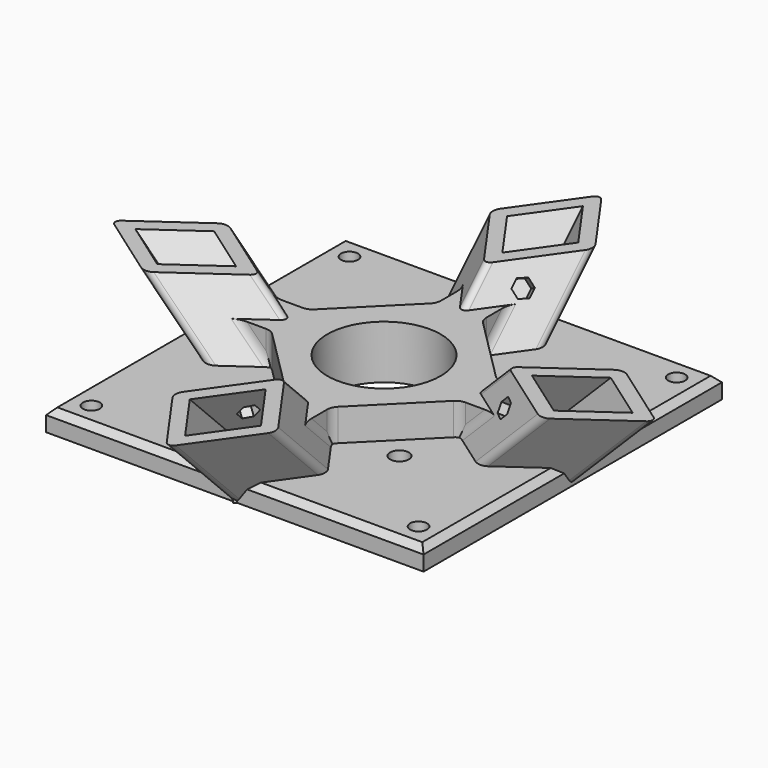
from build123d import *

# Parameters (mm, degrees)
F1_DEPTH      = 4.318
F9_DEPTH      = 2.54
F10_COUNT     = 4
F10_ANGLE     = 270
F14_DEPTH     = 10.795
F23_W         = 111.76
F23_H         = 15.24
F24_DEPTH     = 152.4
F25_T4_DEPTH  = 14.9351248517
F25_T9_DEPTH  = 24.0949860952
F25_T14_DEPTH = 30.2015602576
F25_T19_DEPTH = 30.2015602576
F25_T24_DEPTH = 24.0949860952
F25_T29_DEPTH = 24.0949860952
F25_T34_DEPTH = 30.2015602576
F25_T39_DEPTH = 30.2015602576
F25_T44_DEPTH = 24.0949860952
F25_T49_DEPTH = 14.9351248517
F26_T4_DEPTH  = 24.0949860952
F26_T9_DEPTH  = 30.2015602576
F26_T14_DEPTH = 30.2015602576
F26_T19_DEPTH = 24.0949860952
F26_T24_DEPTH = 14.9351248517
F26_T29_DEPTH = 14.9351248517
F26_T34_DEPTH = 24.0949860952
F26_T39_DEPTH = 24.0949860952
F26_T44_DEPTH = 30.2015602576
F26_T49_DEPTH = 30.2015602576
F27_T1_DEPTH  = 9.1072561211
F27_T6_DEPTH  = 14.4203734854
F27_T11_DEPTH = 14.4203734856
F27_T16_DEPTH = 14.4203734854
F27_T21_DEPTH = 14.4203734856
F27_T26_DEPTH = 14.4203734854
F27_T31_DEPTH = 14.4203734856
F27_T36_DEPTH = 14.4203734856
F27_T41_DEPTH = 14.4203734854
F28_W         = 76.2
F28_H         = 75.2855999997
F29_DEPTH     = 4.318
F15_R         = 1.905
F30_DEPTH     = 25.4
F12_R         = 11.43
F31_DEPTH     = 25.4
F32_R         = 1.7145
F33_DEPTH     = 4.318
F34_SIZE      = 1.27


# Not quite as in the source:
# - a fillet or chamfer that OpenCascade refuses, or shapes differently, is made with other operations: its cross-section is extruded or revolved along the edge and cut away or added


with BuildPart() as f1:
    # F0 (on Top) → F1 (new body)
    with BuildSketch(Plane.XY):
        Polygon((38.1, 0), (0, 38.1), (-38.1, 0), (0, -38.1), align=None)
    extrude(amount=F1_DEPTH)

    # F5 (on offset) → F6 (join, up to the next surface of F1)
    with BuildSketch(Plane(origin=(0, -35.9210244843, 35.9210244843), x_dir=(1, 0, 0), z_dir=(0, 0.7071067812, -0.7071067812))):
        Polygon((10.5607811984, 16.3799871648), (0, 26.9407683632), (-10.5607811984, 16.3799871648), (0, 5.8192059665), align=None)
        Polygon((-7.1842048969, 16.3799871648), (0, 23.5641920617), (7.1842048969, 16.3799871648), (0, 9.195782268), align=None, mode=Mode.SUBTRACT)
    extrude(until=Until.NEXT)

    # F8 (on offset) → F9 (cut)
    with BuildSketch(Plane(origin=(2.9096029833, -2.0574, -2.0574), x_dir=(-0.4082482905, -0.8660254038, 0.2886751346), z_dir=(-0.7071067812, 0.5, 0.5))):
        Polygon((30.7118833173, 5.5090421757), (32.268461045, 6.6097088424), (32.0935446144, 8.5080780308), (30.3620504561, 9.3057805526), (28.8054727285, 8.2051138859), (28.9803891591, 6.3067446975), align=None)
    extrude(amount=-F9_DEPTH, mode=Mode.SUBTRACT)


with BuildPart() as f10_1:
    # F10: instance of F1
    add(f1.part.rotate(Axis((0, 0, 13.9133725866), (0, 0, 1)), 1 * F10_ANGLE / (F10_COUNT - 1)))


with BuildPart() as f10_2:
    # F10: instance of F1
    add(f1.part.rotate(Axis((0, 0, 13.9133725866), (0, 0, 1)), 2 * F10_ANGLE / (F10_COUNT - 1)))


with BuildPart() as f10_3:
    # F10: instance of F1
    add(f1.part.rotate(Axis((0, 0, 13.9133725866), (0, 0, 1)), 3 * F10_ANGLE / (F10_COUNT - 1)))


with BuildPart() as f14:
    # F13 (on Top) → F14 (new body)
    with BuildSketch(Plane.XY):
        Polygon((19.05, 4.597891134), (4.5978911339, 19.05), (-4.5978911339, 19.05), (-19.05, 4.5978911339), (-19.05, -4.597891134), (-4.5978911339, -19.05), (4.597891134, -19.05), (19.05, -4.5978911339), align=None)
    extrude(amount=F14_DEPTH)


with BuildPart() as f10_2_1:
    add(f10_2.part)

    # F16: union F14
    add(f14.part)

    # F17: union F10_3, F1, F10_1
    add(f10_3.part)
    add(f1.part)
    add(f10_1.part)

    # F17_face (on face) → F18 (join, up to the next surface of F10_2)
    with BuildSketch(Plane(origin=(-19.05, 3.0712475933, 8.6360000001), x_dir=(0, -1, 0), z_dir=(-1, 0, 0))):
        Polygon((3.0532870811, 2.1589999999), (-1.5266435405, 2.1589999999), (-1.5266435405, -4.3180000001), align=None)
        Polygon((7.6691387273, -4.3180000001), (7.6691387273, 2.1589999999), (3.0892081056, 2.1589999999), align=None)
    extrude(until=Until.NEXT)

    # F16_face (on face) → F19 (join, up to the next surface of F10_2)
    with BuildSketch(Plane(origin=(-3.0712475933, 19.05, 8.6359999999), x_dir=(-1, 0, 0), z_dir=(0, 1, 0))):
        Polygon((1.5266435406, -4.3179999999), (1.5266435406, 2.1590000001), (-3.0532870811, 2.1590000001), align=None)
        Polygon((-7.6691387272, -4.3179999998), (-3.0892081056, 2.1590000001), (-7.6691387272, 2.1590000001), align=None)
    extrude(until=Until.NEXT)

    # F17_face1 (on face) → F20 (join, up to the next surface of F10_2)
    with BuildSketch(Plane(origin=(19.05, -3.0712475933, 8.6360000001), x_dir=(0, 1, 0), z_dir=(1, 0, 0))):
        Polygon((3.0532870811, 2.1589999999), (-1.5266435405, 2.1589999999), (-1.5266435405, -4.3180000001), align=None)
        Polygon((7.6691387273, -4.3180000001), (7.6691387273, 2.1589999999), (3.0892081056, 2.1589999999), align=None)
    extrude(until=Until.NEXT)

    # F17_face2 (on face) → F21 (join, up to the next surface of F10_2)
    with BuildSketch(Plane(origin=(3.0712475934, -19.05, 8.636), x_dir=(1, 0, 0), z_dir=(0, -1, 0))):
        Polygon((1.5266435406, -4.318), (1.5266435406, 2.159), (-3.0532870811, 2.159), align=None)
        Polygon((-3.0892081056, 2.159), (-7.6691387273, 2.159), (-7.6691387273, -4.318), align=None)
    extrude(until=Until.NEXT)

    # F23 (on offset) → F24 (cut)
    with BuildSketch(Plane.YZ.offset(63.5)):
        with Locations((0, 24.4856)):
            Rectangle(F23_W, F23_H)
    extrude(amount=-F24_DEPTH, mode=Mode.SUBTRACT)

    # F25: fillet of radius 1.27 on 8 edges, made by hand


with BuildPart() as f25_tool2:
    # F25_s3 → F25_t4 (new body)
    with BuildSketch(Plane(origin=(0, 23.2254640303, 23.2254640303), x_dir=(1, 0, 0), z_dir=(0, -0.7071067812, -0.7071067812))):
        with BuildLine():
            ThreePointArc((0.8980256121, -6.7172315786), (0, -6.3452571907), (-0.8980256121, -6.7172315786))
            Line((-0.8980256121, -6.7172315786), (0, -5.8192059665))
            Line((0, -5.8192059665), (0.8980256121, -6.7172315786))
        make_face()
    extrude(amount=F25_T4_DEPTH)

    split(bisect_by=Plane.XY.offset(10.795), keep=Keep.TOP)


with BuildPart() as f10_2_2:
    add(f10_2_1.part)

    # F25_t1: cut F25_tool2
    add(f25_tool2.part, mode=Mode.SUBTRACT)


with BuildPart() as f25_tool7:
    # F25_s8 → F25_t9 (new body)
    with BuildSketch(Plane(origin=(0, 30.6930640303, 30.6930640303), x_dir=(1, 0, 0), z_dir=(0, -0.7071067812, -0.7071067812))):
        with BuildLine():
            ThreePointArc((9.6627555863, -17.2780127769), (10.0347299742, -16.3799871648), (9.6627555863, -15.4819615527))
            Line((9.6627555863, -15.4819615527), (10.5607811984, -16.3799871648))
            Line((10.5607811984, -16.3799871648), (9.6627555863, -17.2780127769))
        make_face()
    extrude(amount=F25_T9_DEPTH)

    split(bisect_by=Plane.XY.offset(4.318), keep=Keep.TOP)


with BuildPart() as f10_2_3:
    add(f10_2_2.part)

    # F25_t6: cut F25_tool7
    add(f25_tool7.part, mode=Mode.SUBTRACT)


with BuildPart() as f25_tool12:
    # F25_s13 → F25_t14 (new body)
    with BuildSketch(Plane(origin=(0, 38.1606640303, 38.1606640303), x_dir=(1, 0, 0), z_dir=(0, -0.7071067812, -0.7071067812))):
        with BuildLine():
            ThreePointArc((0.8980256121, -26.0427427511), (0, -26.414717139), (-0.8980256121, -26.0427427511))
            Line((-0.8980256121, -26.0427427511), (0, -26.9407683632))
            Line((0, -26.9407683632), (0.8980256121, -26.0427427511))
        make_face()
    extrude(amount=F25_T14_DEPTH)

    split(bisect_by=Plane(origin=(-19.05, 19.05, 0), x_dir=(0, 0, 1), z_dir=(-0.7071067812, 0.7071067812, 0)), keep=Keep.TOP)


with BuildPart() as f10_2_4:
    add(f10_2_3.part)

    # F25_t11: cut F25_tool12
    add(f25_tool12.part, mode=Mode.SUBTRACT)


with BuildPart() as f25_tool17:
    # F25_s18 → F25_t19 (new body)
    with BuildSketch(Plane(origin=(0, 38.1606640303, 38.1606640303), x_dir=(1, 0, 0), z_dir=(0, -0.7071067812, -0.7071067812))):
        with BuildLine():
            ThreePointArc((0.8980256121, -26.0427427511), (0, -26.414717139), (-0.8980256121, -26.0427427511))
            Line((-0.8980256121, -26.0427427511), (0, -26.9407683632))
            Line((0, -26.9407683632), (0.8980256121, -26.0427427511))
        make_face()
    extrude(amount=F25_T19_DEPTH)

    split(bisect_by=Plane(origin=(19.05, 19.05, 0), x_dir=(0, 0, 1), z_dir=(0.7071067812, 0.7071067812, 0)), keep=Keep.TOP)


with BuildPart() as f10_2_5:
    add(f10_2_4.part)

    # F25_t16: cut F25_tool17
    add(f25_tool17.part, mode=Mode.SUBTRACT)


with BuildPart() as f25_tool22:
    # F25_s23 → F25_t24 (new body)
    with BuildSketch(Plane(origin=(0, 30.6930640303, 30.6930640303), x_dir=(1, 0, 0), z_dir=(0, -0.7071067812, -0.7071067812))):
        with BuildLine():
            ThreePointArc((-9.6627555863, -17.2780127769), (-10.0347299742, -16.3799871648), (-9.6627555863, -15.4819615527))
            Line((-9.6627555863, -15.4819615527), (-10.5607811984, -16.3799871648))
            Line((-10.5607811984, -16.3799871648), (-9.6627555863, -17.2780127769))
        make_face()
    extrude(amount=F25_T24_DEPTH)

    split(bisect_by=Plane.XY.offset(4.318), keep=Keep.TOP)


with BuildPart() as f10_2_6:
    add(f10_2_5.part)

    # F25_t21: cut F25_tool22
    add(f25_tool22.part, mode=Mode.SUBTRACT)


with BuildPart() as f25_tool27:
    # F25_s28 → F25_t29 (new body)
    with BuildSketch(Plane(origin=(30.6930640303, 0, 30.6930640303), x_dir=(0, 1, 0), z_dir=(-0.7071067812, 0, -0.7071067812))):
        with BuildLine():
            ThreePointArc((9.6627555863, 17.2780127769), (10.0347299742, 16.3799871648), (9.6627555863, 15.4819615527))
            Line((9.6627555863, 15.4819615527), (10.5607811984, 16.3799871648))
            Line((10.5607811984, 16.3799871648), (9.6627555863, 17.2780127769))
        make_face()
    extrude(amount=F25_T29_DEPTH)

    split(bisect_by=Plane.XY.offset(4.318), keep=Keep.TOP)


with BuildPart() as f10_2_7:
    add(f10_2_6.part)

    # F25_t26: cut F25_tool27
    add(f25_tool27.part, mode=Mode.SUBTRACT)


with BuildPart() as f25_tool32:
    # F25_s33 → F25_t34 (new body)
    with BuildSketch(Plane(origin=(38.1606640303, 0, 38.1606640303), x_dir=(0, 1, 0), z_dir=(-0.7071067812, 0, -0.7071067812))):
        with BuildLine():
            ThreePointArc((-0.8980256121, 26.0427427511), (0, 26.414717139), (0.8980256121, 26.0427427511))
            Line((0.8980256121, 26.0427427511), (0, 26.9407683632))
            Line((0, 26.9407683632), (-0.8980256121, 26.0427427511))
        make_face()
    extrude(amount=F25_T34_DEPTH)

    split(bisect_by=Plane(origin=(19.05, 19.05, 0), x_dir=(0, 0, 1), z_dir=(0.7071067812, 0.7071067812, 0)), keep=Keep.TOP)


with BuildPart() as f10_2_8:
    add(f10_2_7.part)

    # F25_t31: cut F25_tool32
    add(f25_tool32.part, mode=Mode.SUBTRACT)


with BuildPart() as f25_tool37:
    # F25_s38 → F25_t39 (new body)
    with BuildSketch(Plane(origin=(38.1606640303, 0, 38.1606640303), x_dir=(0, 1, 0), z_dir=(-0.7071067812, 0, -0.7071067812))):
        with BuildLine():
            ThreePointArc((-0.8980256121, 26.0427427511), (0, 26.414717139), (0.8980256121, 26.0427427511))
            Line((0.8980256121, 26.0427427511), (0, 26.9407683632))
            Line((0, 26.9407683632), (-0.8980256121, 26.0427427511))
        make_face()
    extrude(amount=F25_T39_DEPTH)

    split(bisect_by=Plane(origin=(19.05, -19.05, 0), x_dir=(0, 0, 1), z_dir=(0.7071067812, -0.7071067812, 0)), keep=Keep.TOP)


with BuildPart() as f10_2_9:
    add(f10_2_8.part)

    # F25_t36: cut F25_tool37
    add(f25_tool37.part, mode=Mode.SUBTRACT)


with BuildPart() as f25_tool42:
    # F25_s43 → F25_t44 (new body)
    with BuildSketch(Plane(origin=(30.6930640303, 0, 30.6930640303), x_dir=(0, 1, 0), z_dir=(-0.7071067812, 0, -0.7071067812))):
        with BuildLine():
            ThreePointArc((-9.6627555863, 17.2780127769), (-10.0347299742, 16.3799871648), (-9.6627555863, 15.4819615527))
            Line((-9.6627555863, 15.4819615527), (-10.5607811984, 16.3799871648))
            Line((-10.5607811984, 16.3799871648), (-9.6627555863, 17.2780127769))
        make_face()
    extrude(amount=F25_T44_DEPTH)

    split(bisect_by=Plane.XY.offset(4.318), keep=Keep.TOP)


with BuildPart() as f10_2_10:
    add(f10_2_9.part)

    # F25_t41: cut F25_tool42
    add(f25_tool42.part, mode=Mode.SUBTRACT)


with BuildPart() as f25_tool47:
    # F25_s48 → F25_t49 (new body)
    with BuildSketch(Plane(origin=(23.2254640303, 0, 23.2254640303), x_dir=(0, 1, 0), z_dir=(-0.7071067812, 0, -0.7071067812))):
        with BuildLine():
            ThreePointArc((-0.8980256121, 6.7172315786), (0, 6.3452571907), (0.8980256121, 6.7172315786))
            Line((0.8980256121, 6.7172315786), (0, 5.8192059665))
            Line((0, 5.8192059665), (-0.8980256121, 6.7172315786))
        make_face()
    extrude(amount=F25_T49_DEPTH)

    split(bisect_by=Plane.XY.offset(10.795), keep=Keep.TOP)


with BuildPart() as f10_2_11:
    add(f10_2_10.part)

    # F25_t46: cut F25_tool47
    add(f25_tool47.part, mode=Mode.SUBTRACT)

    # F26: fillet of radius 1.27 on 8 edges, made by hand


with BuildPart() as f26_tool2:
    # F26_s3 → F26_t4 (new body)
    with BuildSketch(Plane(origin=(0, -30.6930640303, 30.6930640303), x_dir=(1, 0, 0), z_dir=(0, 0.7071067812, -0.7071067812))):
        with BuildLine():
            ThreePointArc((-9.6627555863, 17.2780127769), (-10.0347299742, 16.3799871648), (-9.6627555863, 15.4819615527))
            Line((-9.6627555863, 15.4819615527), (-10.5607811984, 16.3799871648))
            Line((-10.5607811984, 16.3799871648), (-9.6627555863, 17.2780127769))
        make_face()
    extrude(amount=F26_T4_DEPTH)

    split(bisect_by=Plane.XY.offset(4.318), keep=Keep.TOP)


with BuildPart() as f10_2_12:
    add(f10_2_11.part)

    # F26_t1: cut F26_tool2
    add(f26_tool2.part, mode=Mode.SUBTRACT)


with BuildPart() as f26_tool7:
    # F26_s8 → F26_t9 (new body)
    with BuildSketch(Plane(origin=(0, -38.1606640303, 38.1606640303), x_dir=(1, 0, 0), z_dir=(0, 0.7071067812, -0.7071067812))):
        with BuildLine():
            ThreePointArc((0.8980256121, 26.0427427511), (0, 26.414717139), (-0.8980256121, 26.0427427511))
            Line((-0.8980256121, 26.0427427511), (0, 26.9407683632))
            Line((0, 26.9407683632), (0.8980256121, 26.0427427511))
        make_face()
    extrude(amount=F26_T9_DEPTH)

    split(bisect_by=Plane(origin=(-19.05, -19.05, 0), x_dir=(0, 0, 1), z_dir=(-0.7071067812, -0.7071067812, 0)), keep=Keep.TOP)


with BuildPart() as f10_2_13:
    add(f10_2_12.part)

    # F26_t6: cut F26_tool7
    add(f26_tool7.part, mode=Mode.SUBTRACT)


with BuildPart() as f26_tool12:
    # F26_s13 → F26_t14 (new body)
    with BuildSketch(Plane(origin=(0, -38.1606640303, 38.1606640303), x_dir=(1, 0, 0), z_dir=(0, 0.7071067812, -0.7071067812))):
        with BuildLine():
            ThreePointArc((0.8980256121, 26.0427427511), (0, 26.414717139), (-0.8980256121, 26.0427427511))
            Line((-0.8980256121, 26.0427427511), (0, 26.9407683632))
            Line((0, 26.9407683632), (0.8980256121, 26.0427427511))
        make_face()
    extrude(amount=F26_T14_DEPTH)

    split(bisect_by=Plane(origin=(19.05, -19.05, 0), x_dir=(0, 0, 1), z_dir=(0.7071067812, -0.7071067812, 0)), keep=Keep.TOP)


with BuildPart() as f10_2_14:
    add(f10_2_13.part)

    # F26_t11: cut F26_tool12
    add(f26_tool12.part, mode=Mode.SUBTRACT)


with BuildPart() as f26_tool17:
    # F26_s18 → F26_t19 (new body)
    with BuildSketch(Plane(origin=(0, -30.6930640303, 30.6930640303), x_dir=(1, 0, 0), z_dir=(0, 0.7071067812, -0.7071067812))):
        with BuildLine():
            ThreePointArc((9.6627555863, 17.2780127769), (10.0347299742, 16.3799871648), (9.6627555863, 15.4819615527))
            Line((9.6627555863, 15.4819615527), (10.5607811984, 16.3799871648))
            Line((10.5607811984, 16.3799871648), (9.6627555863, 17.2780127769))
        make_face()
    extrude(amount=F26_T19_DEPTH)

    split(bisect_by=Plane.XY.offset(4.318), keep=Keep.TOP)


with BuildPart() as f10_2_15:
    add(f10_2_14.part)

    # F26_t16: cut F26_tool17
    add(f26_tool17.part, mode=Mode.SUBTRACT)


with BuildPart() as f26_tool22:
    # F26_s23 → F26_t24 (new body)
    with BuildSketch(Plane(origin=(0, -23.2254640303, 23.2254640303), x_dir=(1, 0, 0), z_dir=(0, 0.7071067812, -0.7071067812))):
        with BuildLine():
            ThreePointArc((0.8980256121, 6.7172315786), (0, 6.3452571907), (-0.8980256121, 6.7172315786))
            Line((-0.8980256121, 6.7172315786), (0, 5.8192059665))
            Line((0, 5.8192059665), (0.8980256121, 6.7172315786))
        make_face()
    extrude(amount=F26_T24_DEPTH)

    split(bisect_by=Plane.XY.offset(10.795), keep=Keep.TOP)


with BuildPart() as f10_2_16:
    add(f10_2_15.part)

    # F26_t21: cut F26_tool22
    add(f26_tool22.part, mode=Mode.SUBTRACT)


with BuildPart() as f26_tool27:
    # F26_s28 → F26_t29 (new body)
    with BuildSketch(Plane(origin=(-23.2254640303, 0, 23.2254640303), x_dir=(0, 1, 0), z_dir=(0.7071067812, 0, -0.7071067812))):
        with BuildLine():
            ThreePointArc((0.8980256121, -6.7172315786), (0, -6.3452571907), (-0.8980256121, -6.7172315786))
            Line((-0.8980256121, -6.7172315786), (0, -5.8192059665))
            Line((0, -5.8192059665), (0.8980256121, -6.7172315786))
        make_face()
    extrude(amount=F26_T29_DEPTH)

    split(bisect_by=Plane.XY.offset(10.795), keep=Keep.TOP)


with BuildPart() as f10_2_17:
    add(f10_2_16.part)

    # F26_t26: cut F26_tool27
    add(f26_tool27.part, mode=Mode.SUBTRACT)


with BuildPart() as f26_tool32:
    # F26_s33 → F26_t34 (new body)
    with BuildSketch(Plane(origin=(-30.6930640303, 0, 30.6930640303), x_dir=(0, 1, 0), z_dir=(0.7071067812, 0, -0.7071067812))):
        with BuildLine():
            ThreePointArc((-9.6627555863, -17.2780127769), (-10.0347299742, -16.3799871648), (-9.6627555863, -15.4819615527))
            Line((-9.6627555863, -15.4819615527), (-10.5607811984, -16.3799871648))
            Line((-10.5607811984, -16.3799871648), (-9.6627555863, -17.2780127769))
        make_face()
    extrude(amount=F26_T34_DEPTH)

    split(bisect_by=Plane.XY.offset(4.318), keep=Keep.TOP)


with BuildPart() as f10_2_18:
    add(f10_2_17.part)

    # F26_t31: cut F26_tool32
    add(f26_tool32.part, mode=Mode.SUBTRACT)


with BuildPart() as f26_tool37:
    # F26_s38 → F26_t39 (new body)
    with BuildSketch(Plane(origin=(-30.6930640303, 0, 30.6930640303), x_dir=(0, 1, 0), z_dir=(0.7071067812, 0, -0.7071067812))):
        with BuildLine():
            ThreePointArc((9.6627555863, -17.2780127769), (10.0347299742, -16.3799871648), (9.6627555863, -15.4819615527))
            Line((9.6627555863, -15.4819615527), (10.5607811984, -16.3799871648))
            Line((10.5607811984, -16.3799871648), (9.6627555863, -17.2780127769))
        make_face()
    extrude(amount=F26_T39_DEPTH)

    split(bisect_by=Plane.XY.offset(4.318), keep=Keep.TOP)


with BuildPart() as f10_2_19:
    add(f10_2_18.part)

    # F26_t36: cut F26_tool37
    add(f26_tool37.part, mode=Mode.SUBTRACT)


with BuildPart() as f26_tool42:
    # F26_s43 → F26_t44 (new body)
    with BuildSketch(Plane(origin=(-38.1606640303, 0, 38.1606640303), x_dir=(0, 1, 0), z_dir=(0.7071067812, 0, -0.7071067812))):
        with BuildLine():
            ThreePointArc((0.8980256121, -26.0427427511), (0, -26.414717139), (-0.8980256121, -26.0427427511))
            Line((-0.8980256121, -26.0427427511), (0, -26.9407683632))
            Line((0, -26.9407683632), (0.8980256121, -26.0427427511))
        make_face()
    extrude(amount=F26_T44_DEPTH)

    split(bisect_by=Plane(origin=(-19.05, -19.05, 0), x_dir=(0, 0, 1), z_dir=(-0.7071067812, -0.7071067812, 0)), keep=Keep.TOP)


with BuildPart() as f10_2_20:
    add(f10_2_19.part)

    # F26_t41: cut F26_tool42
    add(f26_tool42.part, mode=Mode.SUBTRACT)


with BuildPart() as f26_tool47:
    # F26_s48 → F26_t49 (new body)
    with BuildSketch(Plane(origin=(-38.1606640303, 0, 38.1606640303), x_dir=(0, 1, 0), z_dir=(0.7071067812, 0, -0.7071067812))):
        with BuildLine():
            ThreePointArc((0.8980256121, -26.0427427511), (0, -26.414717139), (-0.8980256121, -26.0427427511))
            Line((-0.8980256121, -26.0427427511), (0, -26.9407683632))
            Line((0, -26.9407683632), (0.8980256121, -26.0427427511))
        make_face()
    extrude(amount=F26_T49_DEPTH)

    split(bisect_by=Plane(origin=(-19.05, 19.05, 0), x_dir=(0, 0, 1), z_dir=(-0.7071067812, 0.7071067812, 0)), keep=Keep.TOP)


with BuildPart() as f10_2_21:
    add(f10_2_20.part)

    # F26_t46: cut F26_tool47
    add(f26_tool47.part, mode=Mode.SUBTRACT)

    # F27: fillet of radius 2.54 on 16 edges, made by hand

    # F27_s2 → F27_t1 (join)
    with BuildSketch(Plane.XY.offset(1.6877438789)):
        with BuildLine():
            ThreePointArc((18.3060512242, 5.3418399098), (19.1300865302, 4.7912371214), (20.1021024484, 4.597891134))
            Line((20.1021024484, 4.597891134), (19.05, 4.597891134))
            Line((19.05, 4.597891134), (18.3060512242, 5.3418399098))
        make_face()
        with BuildLine():
            ThreePointArc((4.5978911339, 20.1021024484), (4.7912371213, 19.1300865302), (5.3418399097, 18.3060512242))
            Line((5.3418399097, 18.3060512242), (4.5978911339, 19.05))
            Line((4.5978911339, 19.05), (4.5978911339, 20.1021024484))
        make_face()
        with BuildLine():
            ThreePointArc((-5.3418399097, 18.3060512242), (-4.7912371213, 19.1300865302), (-4.5978911339, 20.1021024484))
            Line((-4.5978911339, 20.1021024484), (-4.5978911339, 19.05))
            Line((-4.5978911339, 19.05), (-5.3418399097, 18.3060512242))
        make_face()
        with BuildLine():
            ThreePointArc((-20.1021024484, 4.5978911339), (-19.1300865302, 4.7912371213), (-18.3060512242, 5.3418399097))
            Line((-18.3060512242, 5.3418399097), (-19.05, 4.5978911339))
            Line((-19.05, 4.5978911339), (-20.1021024484, 4.5978911339))
        make_face()
        with BuildLine():
            ThreePointArc((-18.3060512242, -5.3418399097), (-19.1300865302, -4.7912371214), (-20.1021024484, -4.597891134))
            Line((-20.1021024484, -4.597891134), (-19.05, -4.597891134))
            Line((-19.05, -4.597891134), (-18.3060512242, -5.3418399097))
        make_face()
        with BuildLine():
            ThreePointArc((-4.5978911339, -20.1021024484), (-4.7912371213, -19.1300865302), (-5.3418399097, -18.3060512242))
            Line((-5.3418399097, -18.3060512242), (-4.5978911339, -19.05))
            Line((-4.5978911339, -19.05), (-4.5978911339, -20.1021024484))
        make_face()
        with BuildLine():
            ThreePointArc((4.597891134, -20.1021024484), (4.7912371214, -19.1300865302), (5.3418399097, -18.3060512242))
            Line((5.3418399097, -18.3060512242), (4.597891134, -19.05))
            Line((4.597891134, -19.05), (4.597891134, -20.1021024484))
        make_face()
        with BuildLine():
            ThreePointArc((20.1021024484, -4.5978911339), (19.1300865302, -4.7912371213), (18.3060512242, -5.3418399097))
            Line((18.3060512242, -5.3418399097), (19.05, -4.5978911339))
            Line((19.05, -4.5978911339), (20.1021024484, -4.5978911339))
        make_face()
    extrude(amount=F27_T1_DEPTH)


with BuildPart() as f27_tool4:
    # F27_s5 → F27_t6 (new body)
    with BuildSketch(Plane(origin=(0, -9.8241280606, 9.8241280606), x_dir=(1, 0, 0), z_dir=(0, -0.7071067812, 0.7071067812))):
        with BuildLine():
            ThreePointArc((-5.3418399097, -11.1610458761), (-4.7912371213, -10.3370105701), (-4.5978911339, -9.3649946519))
            Line((-4.5978911339, -9.3649946519), (-4.5978911339, -10.4170971004))
            Line((-4.5978911339, -10.4170971004), (-5.3418399097, -11.1610458761))
        make_face()
    extrude(amount=F27_T6_DEPTH)

    split(bisect_by=Plane.XY.offset(10.795), keep=Keep.BOTTOM)


with BuildPart() as f10_2_22:
    add(f10_2_21.part)

    # F27_t3: union F27_tool4
    add(f27_tool4.part)


with BuildPart() as f27_tool9:
    # F27_s10 → F27_t11 (new body)
    with BuildSketch(Plane(origin=(-20.0208719394, 0, 20.0208719394), x_dir=(0, 1, 0), z_dir=(0.7071067812, 0, -0.7071067812))):
        with BuildLine():
            ThreePointArc((-4.597891134, -9.364994652), (-4.7912371214, -10.3370105702), (-5.3418399097, -11.1610458762))
            Line((-5.3418399097, -11.1610458762), (-4.597891134, -10.4170971004))
            Line((-4.597891134, -10.4170971004), (-4.597891134, -9.364994652))
        make_face()
    extrude(amount=F27_T11_DEPTH)

    split(bisect_by=Plane.XY.offset(10.795), keep=Keep.BOTTOM)


with BuildPart() as f10_2_23:
    add(f10_2_22.part)

    # F27_t8: union F27_tool9
    add(f27_tool9.part)


with BuildPart() as f27_tool14:
    # F27_s15 → F27_t16 (new body)
    with BuildSketch(Plane(origin=(-9.8241280606, 0, 9.8241280606), x_dir=(0, 1, 0), z_dir=(-0.7071067812, 0, 0.7071067812))):
        with BuildLine():
            ThreePointArc((5.3418399097, 11.1610458761), (4.7912371213, 10.3370105701), (4.5978911339, 9.3649946519))
            Line((4.5978911339, 9.3649946519), (4.5978911339, 10.4170971003))
            Line((4.5978911339, 10.4170971003), (5.3418399097, 11.1610458761))
        make_face()
    extrude(amount=F27_T16_DEPTH)

    split(bisect_by=Plane.XY.offset(10.795), keep=Keep.BOTTOM)


with BuildPart() as f10_2_24:
    add(f10_2_23.part)

    # F27_t13: union F27_tool14
    add(f27_tool14.part)


with BuildPart() as f27_tool19:
    # F27_s20 → F27_t21 (new body)
    with BuildSketch(Plane(origin=(0, 20.0208719394, 20.0208719394), x_dir=(1, 0, 0), z_dir=(0, -0.7071067812, -0.7071067812))):
        with BuildLine():
            ThreePointArc((-4.5978911339, -9.364994652), (-4.7912371213, -10.3370105702), (-5.3418399097, -11.1610458762))
            Line((-5.3418399097, -11.1610458762), (-4.5978911339, -10.4170971004))
            Line((-4.5978911339, -10.4170971004), (-4.5978911339, -9.364994652))
        make_face()
    extrude(amount=F27_T21_DEPTH)

    split(bisect_by=Plane.XY.offset(10.795), keep=Keep.BOTTOM)


with BuildPart() as f10_2_25:
    add(f10_2_24.part)

    # F27_t18: union F27_tool19
    add(f27_tool19.part)


with BuildPart() as f27_tool24:
    # F27_s25 → F27_t26 (new body)
    with BuildSketch(Plane(origin=(0, 9.8241280606, 9.8241280606), x_dir=(1, 0, 0), z_dir=(0, 0.7071067812, 0.7071067812))):
        with BuildLine():
            ThreePointArc((5.3418399097, 11.1610458761), (4.7912371213, 10.3370105701), (4.5978911339, 9.3649946519))
            Line((4.5978911339, 9.3649946519), (4.5978911339, 10.4170971004))
            Line((4.5978911339, 10.4170971004), (5.3418399097, 11.1610458761))
        make_face()
    extrude(amount=F27_T26_DEPTH)

    split(bisect_by=Plane.XY.offset(10.795), keep=Keep.BOTTOM)


with BuildPart() as f10_2_26:
    add(f10_2_25.part)

    # F27_t23: union F27_tool24
    add(f27_tool24.part)


with BuildPart() as f27_tool29:
    # F27_s30 → F27_t31 (new body)
    with BuildSketch(Plane(origin=(20.0208719395, 0, 20.0208719395), x_dir=(0, 1, 0), z_dir=(-0.7071067812, 0, -0.7071067812))):
        with BuildLine():
            ThreePointArc((4.597891134, 9.364994652), (4.7912371214, 10.3370105702), (5.3418399098, 11.1610458762))
            Line((5.3418399098, 11.1610458762), (4.597891134, 10.4170971004))
            Line((4.597891134, 10.4170971004), (4.597891134, 9.364994652))
        make_face()
    extrude(amount=F27_T31_DEPTH)

    split(bisect_by=Plane.XY.offset(10.795), keep=Keep.BOTTOM)


with BuildPart() as f10_2_27:
    add(f10_2_26.part)

    # F27_t28: union F27_tool29
    add(f27_tool29.part)


with BuildPart() as f27_tool34:
    # F27_s35 → F27_t36 (new body)
    with BuildSketch(Plane(origin=(0, -20.0208719394, 20.0208719394), x_dir=(1, 0, 0), z_dir=(0, 0.7071067812, -0.7071067812))):
        with BuildLine():
            ThreePointArc((4.597891134, 9.364994652), (4.7912371214, 10.3370105702), (5.3418399097, 11.1610458762))
            Line((5.3418399097, 11.1610458762), (4.597891134, 10.4170971004))
            Line((4.597891134, 10.4170971004), (4.597891134, 9.364994652))
        make_face()
    extrude(amount=F27_T36_DEPTH)

    split(bisect_by=Plane.XY.offset(10.795), keep=Keep.BOTTOM)


with BuildPart() as f10_2_28:
    add(f10_2_27.part)

    # F27_t33: union F27_tool34
    add(f27_tool34.part)


with BuildPart() as f27_tool39:
    # F27_s40 → F27_t41 (new body)
    with BuildSketch(Plane(origin=(9.8241280606, 0, 9.8241280606), x_dir=(0, 1, 0), z_dir=(0.7071067812, 0, 0.7071067812))):
        with BuildLine():
            ThreePointArc((-4.5978911339, -9.3649946519), (-4.7912371213, -10.3370105701), (-5.3418399097, -11.1610458761))
            Line((-5.3418399097, -11.1610458761), (-4.5978911339, -10.4170971003))
            Line((-4.5978911339, -10.4170971003), (-4.5978911339, -9.3649946519))
        make_face()
    extrude(amount=F27_T41_DEPTH)

    split(bisect_by=Plane.XY.offset(10.795), keep=Keep.BOTTOM)


with BuildPart() as f10_2_29:
    add(f10_2_28.part)

    # F27_t38: union F27_tool39
    add(f27_tool39.part)

    # F28 (on Top) → F29 (join)
    with BuildSketch(Plane.XY):
        Rectangle(F28_W, F28_H)
    extrude(amount=F29_DEPTH)

    # F15 (on offset) → F30 (cut)
    with BuildSketch(Plane.XY.offset(25.4)):
        with Locations((-15.6256456507, 15.6256456507)):
            Circle(F15_R)
        with Locations((15.6256456507, 15.6256456507)):
            Circle(F15_R)
        with Locations((15.6256456507, -15.6256456507)):
            Circle(F15_R)
        with Locations((-15.6256456507, -15.6256456507)):
            Circle(F15_R)
    extrude(amount=-F30_DEPTH, mode=Mode.SUBTRACT)

    # F12 (on offset) → F31 (cut)
    with BuildSketch(Plane.XY.offset(25.4)):
        Circle(F12_R)
    extrude(amount=-F31_DEPTH, mode=Mode.SUBTRACT)

    # F32 (on Top) → F33 (cut)
    with BuildSketch(Plane.XY):
        with Locations((-33.02, -32.5627999999)):
            Circle(F32_R)
        with Locations((33.02, -32.5627999999)):
            Circle(F32_R)
        with Locations((33.02, 32.5627999999)):
            Circle(F32_R)
        with Locations((-33.02, 32.5627999999)):
            Circle(F32_R)
    extrude(amount=F33_DEPTH, mode=Mode.SUBTRACT)

    # F34
    f34_edges = [f10_2_29.edges().sort_by_distance(p)[0] for p in [
        (20.738288, -37.6428, 4.318),
        (38.1, -20.348044, 4.318),
        (38.1, 20.348044, 4.318),
        (20.738288, 37.6428, 4.318),
        (-20.738288, 37.6428, 4.318),
        (-38.1, 20.348044, 4.318),
        (-38.1, -20.348044, 4.318),
        (-20.738288, -37.6428, 4.318),
    ]]
    chamfer(f34_edges, length=F34_SIZE)


solid = f10_2_29.part
